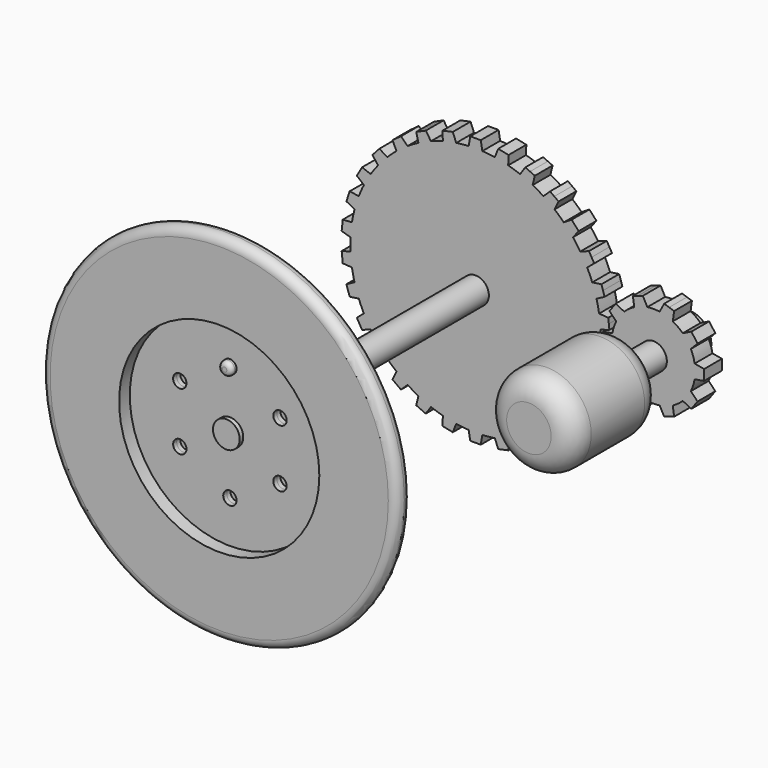
from build123d import *

# Parameters (mm, degrees)
F0_R      = 3
F1_DEPTH  = 80
F0_R_2    = 5
F2_DEPTH  = 5
F3_DEPTH  = 5
F4_DEPTH  = 25
F6_DEPTH  = 5
F8_DEPTH  = 5
F9_R      = 40
F10_DEPTH = 2
F12_R     = 10
F13_DEPTH = 25
F16_R     = 25
F17_DEPTH = 2
F19_R     = 22.5
F20_DEPTH = 3
F21_R     = 1.5
F22_DEPTH = 2
F23_DEPTH = 3.5
F24_R     = 1
F25_R     = 1.99999
F26_R     = 5


# Not quite as in the source:
# - a fillet or chamfer is up to 0.001 mm smaller than in the source, because OpenCascade refuses the exact size
# - a feature of the source that left no trace in its solid (it failed there, or was rolled back) is left out


with BuildPart() as f1:
    # F0 (on Front) → F1 (new body)
    with BuildSketch(Plane.XZ):
        Circle(F0_R)
    extrude(amount=F1_DEPTH)

    # F5 (on face) → F6 (join)
    with BuildSketch(Plane.XZ.offset(5)):
        with BuildLine():
            ThreePointArc((28.0898484802, -1.4057159597), (28.1162107467, -0.7030776964), (28.125, 0))
            ThreePointArc((28.125, 0), (28.1162107467, 0.7030776964), (28.0898484802, 1.4057159597))
            ThreePointArc((28.0898484802, 1.4057159597), (27.9709283072, 2.9398630294), (27.7682826779, 4.4652101991))
            ThreePointArc((27.7682826779, 4.4652101991), (27.5104012706, 5.8475163042), (27.1837531139, 7.2152055856))
            ThreePointArc((27.1837531139, 7.2152055856), (26.7484645208, 8.6911029668), (26.2331096755, 10.1409852457))
            ThreePointArc((26.2331096755, 10.1409852457), (25.6934659962, 11.4394680865), (25.0895972944, 12.709356105))
            ThreePointArc((25.0895972944, 12.709356105), (24.3569644814, 14.0625), (23.5514238999, 15.3735505752))
            ThreePointArc((23.5514238999, 15.3735505752), (22.7536029668, 16.5314602207), (21.8989056799, 17.6480467764))
            ThreePointArc((21.8989056799, 17.6480467764), (20.9009482166, 18.8192983038), (19.8404278876, 19.934217974))
            ThreePointArc((19.8404278876, 19.934217974), (18.8192983038, 20.9009482166), (17.7511268046, 21.815433119))
            ThreePointArc((17.7511268046, 21.815433119), (16.5314602207, 22.7536029668), (15.2623099717, 23.6236643925))
            ThreePointArc((15.2623099717, 23.6236643925), (14.0625, 24.3569644814), (12.8275385085, 25.0293803521))
            ThreePointArc((12.8275385085, 25.0293803521), (11.4394680865, 25.6934659962), (10.0171558733, 26.280643318))
            ThreePointArc((10.0171558733, 26.280643318), (8.6911029668, 26.7484645208), (7.3433252263, 27.1494235596))
            ThreePointArc((7.3433252263, 27.1494235596), (5.8475163042, 27.5104012706), (4.3342039956, 27.7890320221))
            ThreePointArc((4.3342039956, 27.7890320221), (2.9398630294, 27.9709283072), (1.5381733945, 28.0829066802))
            ThreePointArc((1.5381733945, 28.0829066802), (0, 28.125), (-1.5381733945, 28.0829066802))
            ThreePointArc((-1.5381733945, 28.0829066802), (-2.9398630294, 27.9709283072), (-4.3342039956, 27.7890320221))
            ThreePointArc((-4.3342039956, 27.7890320221), (-5.8475163042, 27.5104012706), (-7.3433252263, 27.1494235596))
            ThreePointArc((-7.3433252263, 27.1494235596), (-8.6911029668, 26.7484645208), (-10.0171558733, 26.280643318))
            ThreePointArc((-10.0171558733, 26.280643318), (-11.4394680865, 25.6934659962), (-12.8275385085, 25.0293803521))
            ThreePointArc((-12.8275385085, 25.0293803521), (-14.0625, 24.3569644814), (-15.2623099717, 23.6236643925))
            ThreePointArc((-15.2623099717, 23.6236643925), (-16.5314602207, 22.7536029668), (-17.7511268046, 21.815433119))
            ThreePointArc((-17.7511268046, 21.815433119), (-18.8192983038, 20.9009482166), (-19.8404278876, 19.934217974))
            ThreePointArc((-19.8404278876, 19.934217974), (-20.9009482166, 18.8192983038), (-21.8989056799, 17.6480467764))
            ThreePointArc((-21.8989056799, 17.6480467764), (-22.7536029668, 16.5314602207), (-23.5514238999, 15.3735505752))
            ThreePointArc((-23.5514238999, 15.3735505752), (-24.3569644814, 14.0625), (-25.0895972944, 12.709356105))
            ThreePointArc((-25.0895972944, 12.709356105), (-25.6934659962, 11.4394680865), (-26.2331096755, 10.1409852457))
            ThreePointArc((-26.2331096755, 10.1409852457), (-26.7484645208, 8.6911029668), (-27.1837531139, 7.2152055856))
            ThreePointArc((-27.1837531139, 7.2152055856), (-27.5104012706, 5.8475163042), (-27.7682826779, 4.4652101991))
            ThreePointArc((-27.7682826779, 4.4652101991), (-27.9709283072, 2.9398630294), (-28.0898484802, 1.4057159597))
            ThreePointArc((-28.0898484802, 1.4057159597), (-28.125, 0), (-28.0898484802, -1.4057159597))
            ThreePointArc((-28.0898484802, -1.4057159597), (-27.9709283072, -2.9398630294), (-27.7682826779, -4.4652101991))
            ThreePointArc((-27.7682826779, -4.4652101991), (-27.5104012706, -5.8475163042), (-27.1837531139, -7.2152055856))
            ThreePointArc((-27.1837531139, -7.2152055856), (-26.7484645208, -8.6911029668), (-26.2331096755, -10.1409852457))
            ThreePointArc((-26.2331096755, -10.1409852457), (-25.6934659962, -11.4394680865), (-25.0895972944, -12.709356105))
            ThreePointArc((-25.0895972944, -12.709356105), (-24.3569644814, -14.0625), (-23.5514238999, -15.3735505752))
            ThreePointArc((-23.5514238999, -15.3735505752), (-22.7536029668, -16.5314602207), (-21.8989056799, -17.6480467764))
            ThreePointArc((-21.8989056799, -17.6480467764), (-20.9009482166, -18.8192983038), (-19.8404278876, -19.934217974))
            ThreePointArc((-19.8404278876, -19.934217974), (-18.8192983038, -20.9009482166), (-17.7511268046, -21.815433119))
            ThreePointArc((-17.7511268046, -21.815433119), (-16.5314602207, -22.7536029668), (-15.2623099717, -23.6236643925))
            ThreePointArc((-15.2623099717, -23.6236643925), (-14.0625, -24.3569644814), (-12.8275385085, -25.0293803521))
            ThreePointArc((-12.8275385085, -25.0293803521), (-11.4394680865, -25.6934659962), (-10.0171558733, -26.280643318))
            ThreePointArc((-10.0171558733, -26.280643318), (-8.6911029668, -26.7484645208), (-7.3433252263, -27.1494235596))
            ThreePointArc((-7.3433252263, -27.1494235596), (-5.8475163042, -27.5104012706), (-4.3342039956, -27.7890320221))
            ThreePointArc((-4.3342039956, -27.7890320221), (-2.9398630294, -27.9709283072), (-1.5381733945, -28.0829066802))
            ThreePointArc((-1.5381733945, -28.0829066802), (0, -28.125), (1.5381733945, -28.0829066802))
            ThreePointArc((1.5381733945, -28.0829066802), (2.9398630294, -27.9709283072), (4.3342039956, -27.7890320221))
            ThreePointArc((4.3342039956, -27.7890320221), (5.8475163042, -27.5104012706), (7.3433252263, -27.1494235596))
            ThreePointArc((7.3433252263, -27.1494235596), (8.6911029668, -26.7484645208), (10.0171558733, -26.280643318))
            ThreePointArc((10.0171558733, -26.280643318), (11.4394680865, -25.6934659962), (12.8275385085, -25.0293803521))
            ThreePointArc((12.8275385085, -25.0293803521), (14.0625, -24.3569644814), (15.2623099717, -23.6236643925))
            ThreePointArc((15.2623099717, -23.6236643925), (16.5314602207, -22.7536029668), (17.7511268046, -21.815433119))
            ThreePointArc((17.7511268046, -21.815433119), (18.8192983038, -20.9009482166), (19.8404278876, -19.934217974))
            ThreePointArc((19.8404278876, -19.934217974), (20.9009482166, -18.8192983038), (21.8989056799, -17.6480467764))
            ThreePointArc((21.8989056799, -17.6480467764), (22.7536029668, -16.5314602207), (23.5514238999, -15.3735505752))
            ThreePointArc((23.5514238999, -15.3735505752), (24.3569644814, -14.0625), (25.0895972944, -12.709356105))
            ThreePointArc((25.0895972944, -12.709356105), (25.6934659962, -11.4394680865), (26.2331096755, -10.1409852457))
            ThreePointArc((26.2331096755, -10.1409852457), (26.7484645208, -8.6911029668), (27.1837531139, -7.2152055856))
            ThreePointArc((27.1837531139, -7.2152055856), (27.5104012706, -5.8475163042), (27.7682826779, -4.4652101991))
            ThreePointArc((27.7682826779, -4.4652101991), (27.9709283072, -2.9398630294), (28.0898484802, -1.4057159597))
        make_face()
        with BuildLine():
            ThreePointArc((27.7682826779, 4.4652101991), (27.9709283072, 2.9398630294), (28.0898484802, 1.4057159597))
            Line((28.0898484802, 1.4057159597), (30.0831167926, 1.9772764508))
            Line((30.0831167926, 1.9772764508), (29.959972098, 3.1489199559))
            Line((29.959972098, 3.1489199559), (29.8368274034, 4.3205634611))
            Line((29.8368274034, 4.3205634611), (27.7682826779, 4.4652101991))
        make_face()
        with BuildLine():
            Line((30.0831167926, -1.9772764508), (28.0898484802, -1.4057159597))
            ThreePointArc((28.0898484802, -1.4057159597), (27.9709283072, -2.9398630294), (27.7682826779, -4.4652101991))
            Line((27.7682826779, -4.4652101991), (29.8368274034, -4.3205634611))
            Line((29.8368274034, -4.3205634611), (29.959972098, -3.1489199559))
            Line((29.959972098, -3.1489199559), (30.0831167926, -1.9772764508))
        make_face()
        with BuildLine():
            ThreePointArc((26.2331096755, 10.1409852457), (26.7484645208, 8.6911029668), (27.1837531139, 7.2152055856))
            Line((27.1837531139, 7.2152055856), (29.0146296232, 8.1886998938))
            Line((29.0146296232, 8.1886998938), (28.6505775534, 9.3091369555))
            Line((28.6505775534, 9.3091369555), (28.2865254836, 10.4295740173))
            Line((28.2865254836, 10.4295740173), (26.2331096755, 10.1409852457))
        make_face()
        with BuildLine():
            Line((29.0146296232, -8.1886998938), (27.1837531139, -7.2152055856))
            ThreePointArc((27.1837531139, -7.2152055856), (26.7484645208, -8.6911029668), (26.2331096755, -10.1409852457))
            Line((26.2331096755, -10.1409852457), (28.2865254836, -10.4295740173))
            Line((28.2865254836, -10.4295740173), (28.6505775534, -9.3091369555))
            Line((28.6505775534, -9.3091369555), (29.0146296232, -8.1886998938))
        make_face()
        with BuildLine():
            ThreePointArc((23.5514238999, 15.3735505752), (24.3569644814, 14.0625), (25.0895972944, 12.709356105))
            Line((25.0895972944, 12.709356105), (26.6780639116, 14.0422378576))
            Line((26.6780639116, 14.0422378576), (26.089015289, 15.0625))
            Line((26.089015289, 15.0625), (25.4999666665, 16.0827621424))
            Line((25.4999666665, 16.0827621424), (23.5514238999, 15.3735505752))
        make_face()
        with BuildLine():
            Line((26.6780639116, -14.0422378576), (25.0895972944, -12.709356105))
            ThreePointArc((25.0895972944, -12.709356105), (24.3569644814, -14.0625), (23.5514238999, -15.3735505752))
            Line((23.5514238999, -15.3735505752), (25.4999666665, -16.0827621424))
            Line((25.4999666665, -16.0827621424), (26.089015289, -15.0625))
            Line((26.089015289, -15.0625), (26.6780639116, -14.0422378576))
        make_face()
        with BuildLine():
            ThreePointArc((19.8404278876, 19.934217974), (20.9009482166, 18.8192983038), (21.8989056799, 17.6480467764))
            Line((21.8989056799, 17.6480467764), (23.1755387915, 19.282062645))
            Line((23.1755387915, 19.282062645), (22.3872378675, 20.1575595166))
            Line((22.3872378675, 20.1575595166), (21.5989369435, 21.0330563882))
            Line((21.5989369435, 21.0330563882), (19.8404278876, 19.934217974))
        make_face()
        with BuildLine():
            Line((23.1755387915, -19.282062645), (21.8989056799, -17.6480467764))
            ThreePointArc((21.8989056799, -17.6480467764), (20.9009482166, -18.8192983038), (19.8404278876, -19.934217974))
            Line((19.8404278876, -19.934217974), (21.5989369435, -21.0330563882))
            Line((21.5989369435, -21.0330563882), (22.3872378675, -20.1575595166))
            Line((22.3872378675, -20.1575595166), (23.1755387915, -19.282062645))
        make_face()
        with BuildLine():
            ThreePointArc((15.2623099717, 23.6236643925), (16.5314602207, 22.7536029668), (17.7511268046, 21.815433119))
            Line((17.7511268046, 21.815433119), (18.6601314176, 23.6791687691))
            Line((18.6601314176, 23.6791687691), (17.7070307253, 24.3716369555))
            Line((17.7070307253, 24.3716369555), (16.753930033, 25.064105142))
            Line((16.753930033, 25.064105142), (15.2623099717, 23.6236643925))
        make_face()
        with BuildLine():
            Line((18.6601314176, -23.6791687691), (17.7511268046, -21.815433119))
            ThreePointArc((17.7511268046, -21.815433119), (16.5314602207, -22.7536029668), (15.2623099717, -23.6236643925))
            Line((15.2623099717, -23.6236643925), (16.753930033, -25.064105142))
            Line((16.753930033, -25.064105142), (17.7070307253, -24.3716369555))
            Line((17.7070307253, -24.3716369555), (18.6601314176, -23.6791687691))
        make_face()
        with BuildLine():
            ThreePointArc((10.0171558733, 26.280643318), (11.4394680865, 25.6934659962), (12.8275385085, 25.0293803521))
            Line((12.8275385085, 25.0293803521), (13.3291867596, 27.0413815928))
            Line((13.3291867596, 27.0413815928), (12.2529413727, 27.5205569115))
            Line((12.2529413727, 27.5205569115), (11.1766959857, 27.9997322302))
            Line((11.1766959857, 27.9997322302), (10.0171558733, 26.280643318))
        make_face()
        with BuildLine():
            Line((13.3291867596, -27.0413815928), (12.8275385085, -25.0293803521))
            ThreePointArc((12.8275385085, -25.0293803521), (11.4394680865, -25.6934659962), (10.0171558733, -26.280643318))
            Line((10.0171558733, -26.280643318), (11.1766959857, -27.9997322302))
            Line((11.1766959857, -27.9997322302), (12.2529413727, -27.5205569115))
            Line((12.2529413727, -27.5205569115), (13.3291867596, -27.0413815928))
        make_face()
        with BuildLine():
            ThreePointArc((4.3342039956, 27.7890320221), (5.8475163042, 27.5104012706), (7.3433252263, 27.1494235596))
            Line((7.3433252263, 27.1494235596), (7.4156926796, 29.2217562819))
            Line((7.4156926796, 29.2217562819), (6.2633396859, 29.4666964721))
            Line((6.2633396859, 29.4666964721), (5.1109866922, 29.7116366623))
            Line((5.1109866922, 29.7116366623), (4.3342039956, 27.7890320221))
        make_face()
        with BuildLine():
            Line((7.4156926796, -29.2217562819), (7.3433252263, -27.1494235596))
            ThreePointArc((7.3433252263, -27.1494235596), (5.8475163042, -27.5104012706), (4.3342039956, -27.7890320221))
            Line((4.3342039956, -27.7890320221), (5.1109866922, -29.7116366623))
            Line((5.1109866922, -29.7116366623), (6.2633396859, -29.4666964721))
            Line((6.2633396859, -29.4666964721), (7.4156926796, -29.2217562819))
        make_face()
        with BuildLine():
            ThreePointArc((-1.5381733945, 28.0829066802), (0, 28.125), (1.5381733945, 28.0829066802))
            Line((1.5381733945, 28.0829066802), (1.1780972451, 30.125))
            Line((1.1780972451, 30.125), (0, 30.125))
            Line((0, 30.125), (-1.1780972451, 30.125))
            Line((-1.1780972451, 30.125), (-1.5381733945, 28.0829066802))
        make_face()
        with BuildLine():
            Line((1.1780972451, -30.125), (1.5381733945, -28.0829066802))
            ThreePointArc((1.5381733945, -28.0829066802), (0, -28.125), (-1.5381733945, -28.0829066802))
            Line((-1.5381733945, -28.0829066802), (-1.1780972451, -30.125))
            Line((-1.1780972451, -30.125), (0, -30.125))
            Line((0, -30.125), (1.1780972451, -30.125))
        make_face()
        with BuildLine():
            ThreePointArc((-7.3433252263, 27.1494235596), (-5.8475163042, 27.5104012706), (-4.3342039956, 27.7890320221))
            Line((-4.3342039956, 27.7890320221), (-5.1109866922, 29.7116366623))
            Line((-5.1109866922, 29.7116366623), (-6.2633396859, 29.4666964721))
            Line((-6.2633396859, 29.4666964721), (-7.4156926796, 29.2217562819))
            Line((-7.4156926796, 29.2217562819), (-7.3433252263, 27.1494235596))
        make_face()
        with BuildLine():
            Line((-5.1109866922, -29.7116366623), (-4.3342039956, -27.7890320221))
            ThreePointArc((-4.3342039956, -27.7890320221), (-5.8475163042, -27.5104012706), (-7.3433252263, -27.1494235596))
            Line((-7.3433252263, -27.1494235596), (-7.4156926796, -29.2217562819))
            Line((-7.4156926796, -29.2217562819), (-6.2633396859, -29.4666964721))
            Line((-6.2633396859, -29.4666964721), (-5.1109866922, -29.7116366623))
        make_face()
        with BuildLine():
            ThreePointArc((-12.8275385085, 25.0293803521), (-11.4394680865, 25.6934659962), (-10.0171558733, 26.280643318))
            Line((-10.0171558733, 26.280643318), (-11.1766959857, 27.9997322302))
            Line((-11.1766959857, 27.9997322302), (-12.2529413727, 27.5205569115))
            Line((-12.2529413727, 27.5205569115), (-13.3291867596, 27.0413815928))
            Line((-13.3291867596, 27.0413815928), (-12.8275385085, 25.0293803521))
        make_face()
        with BuildLine():
            Line((-11.1766959857, -27.9997322302), (-10.0171558733, -26.280643318))
            ThreePointArc((-10.0171558733, -26.280643318), (-11.4394680865, -25.6934659962), (-12.8275385085, -25.0293803521))
            Line((-12.8275385085, -25.0293803521), (-13.3291867596, -27.0413815928))
            Line((-13.3291867596, -27.0413815928), (-12.2529413727, -27.5205569115))
            Line((-12.2529413727, -27.5205569115), (-11.1766959857, -27.9997322302))
        make_face()
        with BuildLine():
            ThreePointArc((-17.7511268046, 21.815433119), (-16.5314602207, 22.7536029668), (-15.2623099717, 23.6236643925))
            Line((-15.2623099717, 23.6236643925), (-16.753930033, 25.064105142))
            Line((-16.753930033, 25.064105142), (-17.7070307253, 24.3716369555))
            Line((-17.7070307253, 24.3716369555), (-18.6601314176, 23.6791687691))
            Line((-18.6601314176, 23.6791687691), (-17.7511268046, 21.815433119))
        make_face()
        with BuildLine():
            Line((-16.753930033, -25.064105142), (-15.2623099717, -23.6236643925))
            ThreePointArc((-15.2623099717, -23.6236643925), (-16.5314602207, -22.7536029668), (-17.7511268046, -21.815433119))
            Line((-17.7511268046, -21.815433119), (-18.6601314176, -23.6791687691))
            Line((-18.6601314176, -23.6791687691), (-17.7070307253, -24.3716369555))
            Line((-17.7070307253, -24.3716369555), (-16.753930033, -25.064105142))
        make_face()
        with BuildLine():
            ThreePointArc((-21.8989056799, 17.6480467764), (-20.9009482166, 18.8192983038), (-19.8404278876, 19.934217974))
            Line((-19.8404278876, 19.934217974), (-21.5989369435, 21.0330563882))
            Line((-21.5989369435, 21.0330563882), (-22.3872378675, 20.1575595166))
            Line((-22.3872378675, 20.1575595166), (-23.1755387915, 19.282062645))
            Line((-23.1755387915, 19.282062645), (-21.8989056799, 17.6480467764))
        make_face()
        with BuildLine():
            Line((-21.5989369435, -21.0330563882), (-19.8404278876, -19.934217974))
            ThreePointArc((-19.8404278876, -19.934217974), (-20.9009482166, -18.8192983038), (-21.8989056799, -17.6480467764))
            Line((-21.8989056799, -17.6480467764), (-23.1755387915, -19.282062645))
            Line((-23.1755387915, -19.282062645), (-22.3872378675, -20.1575595166))
            Line((-22.3872378675, -20.1575595166), (-21.5989369435, -21.0330563882))
        make_face()
        with BuildLine():
            ThreePointArc((-25.0895972944, 12.709356105), (-24.3569644814, 14.0625), (-23.5514238999, 15.3735505752))
            Line((-23.5514238999, 15.3735505752), (-25.4999666665, 16.0827621424))
            Line((-25.4999666665, 16.0827621424), (-26.089015289, 15.0625))
            Line((-26.089015289, 15.0625), (-26.6780639116, 14.0422378576))
            Line((-26.6780639116, 14.0422378576), (-25.0895972944, 12.709356105))
        make_face()
        with BuildLine():
            Line((-25.4999666665, -16.0827621424), (-23.5514238999, -15.3735505752))
            ThreePointArc((-23.5514238999, -15.3735505752), (-24.3569644814, -14.0625), (-25.0895972944, -12.709356105))
            Line((-25.0895972944, -12.709356105), (-26.6780639116, -14.0422378576))
            Line((-26.6780639116, -14.0422378576), (-26.089015289, -15.0625))
            Line((-26.089015289, -15.0625), (-25.4999666665, -16.0827621424))
        make_face()
        with BuildLine():
            ThreePointArc((-27.1837531139, 7.2152055856), (-26.7484645208, 8.6911029668), (-26.2331096755, 10.1409852457))
            Line((-26.2331096755, 10.1409852457), (-28.2865254836, 10.4295740173))
            Line((-28.2865254836, 10.4295740173), (-28.6505775534, 9.3091369555))
            Line((-28.6505775534, 9.3091369555), (-29.0146296232, 8.1886998938))
            Line((-29.0146296232, 8.1886998938), (-27.1837531139, 7.2152055856))
        make_face()
        with BuildLine():
            Line((-28.2865254836, -10.4295740173), (-26.2331096755, -10.1409852457))
            ThreePointArc((-26.2331096755, -10.1409852457), (-26.7484645208, -8.6911029668), (-27.1837531139, -7.2152055856))
            Line((-27.1837531139, -7.2152055856), (-29.0146296232, -8.1886998938))
            Line((-29.0146296232, -8.1886998938), (-28.6505775534, -9.3091369555))
            Line((-28.6505775534, -9.3091369555), (-28.2865254836, -10.4295740173))
        make_face()
        with BuildLine():
            ThreePointArc((-28.0898484802, 1.4057159597), (-27.9709283072, 2.9398630294), (-27.7682826779, 4.4652101991))
            Line((-27.7682826779, 4.4652101991), (-29.8368274034, 4.3205634611))
            Line((-29.8368274034, 4.3205634611), (-29.959972098, 3.1489199559))
            Line((-29.959972098, 3.1489199559), (-30.0831167926, 1.9772764508))
            Line((-30.0831167926, 1.9772764508), (-28.0898484802, 1.4057159597))
        make_face()
        with BuildLine():
            Line((-29.8368274034, -4.3205634611), (-27.7682826779, -4.4652101991))
            ThreePointArc((-27.7682826779, -4.4652101991), (-27.9709283072, -2.9398630294), (-28.0898484802, -1.4057159597))
            Line((-28.0898484802, -1.4057159597), (-30.0831167926, -1.9772764508))
            Line((-30.0831167926, -1.9772764508), (-29.959972098, -3.1489199559))
            Line((-29.959972098, -3.1489199559), (-29.8368274034, -4.3205634611))
        make_face()
    extrude(amount=F6_DEPTH)


with BuildPart() as f2:
    # F0 (on Front) → F2 (new body)
    with BuildSketch(Plane.XZ):
        Circle(F0_R_2)
        Circle(F0_R, mode=Mode.SUBTRACT)
    extrude(amount=F2_DEPTH)


with BuildPart() as f3:
    # F0 (on Front) → F3 (new body)
    with BuildSketch(Plane.XZ):
        with Locations((40, 0)):
            Circle(F0_R_2)
        with Locations((40, 0)):
            Circle(F0_R, mode=Mode.SUBTRACT)
    extrude(amount=F3_DEPTH)


with BuildPart() as f4:
    # F0 (on Front) → F4 (new body)
    with BuildSketch(Plane.XZ):
        with Locations((40, 0)):
            Circle(F0_R)
    extrude(amount=F4_DEPTH)

    # F7 (on face) → F8 (join)
    with BuildSketch(Plane.XZ.offset(5)):
        with BuildLine():
            ThreePointArc((49.2453733036, -1.5536078905), (49.3425371212, -0.7795031363), (49.375, 0))
            ThreePointArc((49.375, 0), (49.3425371212, 0.7795031363), (49.2453733036, 1.5536078905))
            ThreePointArc((49.2453733036, 1.5536078905), (48.9161548403, 2.8970343223), (48.3928519278, 4.1773988938))
            ThreePointArc((48.3928519278, 4.1773988938), (47.5845343223, 5.5104867402), (46.566476316, 6.6911892658))
            ThreePointArc((46.566476316, 6.6911892658), (45.5104867402, 7.5845343223), (44.3345463782, 8.3127812852))
            ThreePointArc((44.3345463782, 8.3127812852), (42.8970343223, 8.9161548403), (41.3794085621, 9.2729637667))
            ThreePointArc((41.3794085621, 9.2729637667), (40, 9.375), (38.6205914379, 9.2729637667))
            ThreePointArc((38.6205914379, 9.2729637667), (37.1029656777, 8.9161548403), (35.6654536218, 8.3127812852))
            ThreePointArc((35.6654536218, 8.3127812852), (34.4895132598, 7.5845343223), (33.433523684, 6.6911892658))
            ThreePointArc((33.433523684, 6.6911892658), (32.4154656777, 5.5104867402), (31.6071480722, 4.1773988938))
            ThreePointArc((31.6071480722, 4.1773988938), (31.0838451597, 2.8970343223), (30.7546266964, 1.5536078905))
            ThreePointArc((30.7546266964, 1.5536078905), (30.625, 0), (30.7546266964, -1.5536078905))
            ThreePointArc((30.7546266964, -1.5536078905), (31.0838451597, -2.8970343223), (31.6071480722, -4.1773988938))
            ThreePointArc((31.6071480722, -4.1773988938), (32.4154656777, -5.5104867402), (33.433523684, -6.6911892658))
            ThreePointArc((33.433523684, -6.6911892658), (34.4895132598, -7.5845343223), (35.6654536218, -8.3127812852))
            ThreePointArc((35.6654536218, -8.3127812852), (37.1029656777, -8.9161548403), (38.6205914379, -9.2729637667))
            ThreePointArc((38.6205914379, -9.2729637667), (40, -9.375), (41.3794085621, -9.2729637667))
            ThreePointArc((41.3794085621, -9.2729637667), (42.8970343223, -8.9161548403), (44.3345463782, -8.3127812852))
            ThreePointArc((44.3345463782, -8.3127812852), (45.5104867402, -7.5845343223), (46.566476316, -6.6911892658))
            ThreePointArc((46.566476316, -6.6911892658), (47.5845343223, -5.5104867402), (48.3928519278, -4.1773988938))
            ThreePointArc((48.3928519278, -4.1773988938), (48.9161548403, -2.8970343223), (49.2453733036, -1.5536078905))
        make_face()
        with BuildLine():
            ThreePointArc((49.2453733036, 1.5536078905), (49.3425371212, 0.7795031363), (49.375, 0))
            ThreePointArc((49.375, 0), (49.3425371212, -0.7795031363), (49.2453733036, -1.5536078905))
            Line((49.2453733036, -1.5536078905), (51.375, -1.1780972451))
            Line((51.375, -1.1780972451), (51.375, 0))
            Line((51.375, 0), (51.375, 1.1780972451))
            Line((51.375, 1.1780972451), (49.2453733036, 1.5536078905))
        make_face()
        with BuildLine():
            ThreePointArc((46.566476316, 6.6911892658), (47.5845343223, 5.5104867402), (48.3928519278, 4.1773988938))
            Line((48.3928519278, 4.1773988938), (49.8950364974, 5.7329565525))
            Line((49.8950364974, 5.7329565525), (49.202568311, 6.6860572448))
            Line((49.202568311, 6.6860572448), (48.5101001246, 7.6391579371))
            Line((48.5101001246, 7.6391579371), (46.566476316, 6.6911892658))
        make_face()
        with BuildLine():
            Line((49.8950364974, -5.7329565525), (48.3928519278, -4.1773988938))
            ThreePointArc((48.3928519278, -4.1773988938), (47.5845343223, -5.5104867402), (46.566476316, -6.6911892658))
            Line((46.566476316, -6.6911892658), (48.5101001246, -7.6391579371))
            Line((48.5101001246, -7.6391579371), (49.202568311, -6.6860572448))
            Line((49.202568311, -6.6860572448), (49.8950364974, -5.7329565525))
        make_face()
        with BuildLine():
            ThreePointArc((41.3794085621, 9.2729637667), (42.8970343223, 8.9161548403), (44.3345463782, 8.3127812852))
            Line((44.3345463782, 8.3127812852), (44.6355053728, 10.4542158031))
            Line((44.6355053728, 10.4542158031), (43.515068311, 10.8182678729))
            Line((43.515068311, 10.8182678729), (42.3946312492, 11.1823199426))
            Line((42.3946312492, 11.1823199426), (41.3794085621, 9.2729637667))
        make_face()
        with BuildLine():
            Line((44.6355053728, -10.4542158031), (44.3345463782, -8.3127812852))
            ThreePointArc((44.3345463782, -8.3127812852), (42.8970343223, -8.9161548403), (41.3794085621, -9.2729637667))
            Line((41.3794085621, -9.2729637667), (42.3946312492, -11.1823199426))
            Line((42.3946312492, -11.1823199426), (43.515068311, -10.8182678729))
            Line((43.515068311, -10.8182678729), (44.6355053728, -10.4542158031))
        make_face()
        with BuildLine():
            ThreePointArc((35.6654536218, 8.3127812852), (37.1029656777, 8.9161548403), (38.6205914379, 9.2729637667))
            Line((38.6205914379, 9.2729637667), (37.6053687508, 11.1823199426))
            Line((37.6053687508, 11.1823199426), (36.484931689, 10.8182678729))
            Line((36.484931689, 10.8182678729), (35.3644946272, 10.4542158031))
            Line((35.3644946272, 10.4542158031), (35.6654536218, 8.3127812852))
        make_face()
        with BuildLine():
            Line((37.6053687508, -11.1823199426), (38.6205914379, -9.2729637667))
            ThreePointArc((38.6205914379, -9.2729637667), (37.1029656777, -8.9161548403), (35.6654536218, -8.3127812852))
            Line((35.6654536218, -8.3127812852), (35.3644946272, -10.4542158031))
            Line((35.3644946272, -10.4542158031), (36.484931689, -10.8182678729))
            Line((36.484931689, -10.8182678729), (37.6053687508, -11.1823199426))
        make_face()
        with BuildLine():
            ThreePointArc((31.6071480722, 4.1773988938), (32.4154656777, 5.5104867402), (33.433523684, 6.6911892658))
            Line((33.433523684, 6.6911892658), (31.4898998754, 7.6391579371))
            Line((31.4898998754, 7.6391579371), (30.797431689, 6.6860572448))
            Line((30.797431689, 6.6860572448), (30.1049635026, 5.7329565525))
            Line((30.1049635026, 5.7329565525), (31.6071480722, 4.1773988938))
        make_face()
        with BuildLine():
            Line((31.4898998754, -7.6391579371), (33.433523684, -6.6911892658))
            ThreePointArc((33.433523684, -6.6911892658), (32.4154656777, -5.5104867402), (31.6071480722, -4.1773988938))
            Line((31.6071480722, -4.1773988938), (30.1049635026, -5.7329565525))
            Line((30.1049635026, -5.7329565525), (30.797431689, -6.6860572448))
            Line((30.797431689, -6.6860572448), (31.4898998754, -7.6391579371))
        make_face()
        with BuildLine():
            ThreePointArc((30.7546266964, -1.5536078905), (30.625, 0), (30.7546266964, 1.5536078905))
            Line((30.7546266964, 1.5536078905), (28.625, 1.1780972451))
            Line((28.625, 1.1780972451), (28.625, 0))
            Line((28.625, 0), (28.625, -1.1780972451))
            Line((28.625, -1.1780972451), (30.7546266964, -1.5536078905))
        make_face()
    extrude(amount=F8_DEPTH)


with BuildPart() as f10:
    # F9 (on face) → F10 (new body, symmetric)
    with BuildSketch(Plane.XZ.offset(80)):
        Circle(F9_R)
    extrude(amount=F10_DEPTH, both=True)

    # F11: cut F1
    add(f1.part, mode=Mode.SUBTRACT)

    # F19 (on face) → F20 (cut)
    with BuildSketch(Plane.XZ.offset(82)):
        Circle(F19_R)
    extrude(amount=-F20_DEPTH, mode=Mode.SUBTRACT)


with BuildPart() as f13:
    # F12 (on face) → F13 (new body)
    with BuildSketch(Plane.XZ.offset(25)):
        with Locations((40, 0)):
            Circle(F12_R)
    extrude(amount=F13_DEPTH)


with BuildPart() as f13_1:
    # F14: moved
    add(f13.part.moved(Location((0, 5, 0))))

    # F15: cut F4
    add(f4.part, mode=Mode.SUBTRACT)

    # F26
    f26_edges = [f13_1.edges().sort_by_distance(p)[0] for p in [
        (30, -45, 0),
        (30, -20, 0),
    ]]
    fillet(f26_edges, radius=F26_R)


with BuildPart() as f17:
    # F16 (on face) → F17 (new body)
    with BuildSketch(Plane(origin=(0, -78, 0), x_dir=(-1, 0, 0), z_dir=(0, 1, 0))):
        Circle(F16_R)
    extrude(amount=F17_DEPTH)

    # F18: cut F1
    add(f1.part, mode=Mode.SUBTRACT)


with BuildPart() as f22_tool:
    # F21 (on face) → F22 (new body)
    with BuildSketch(Plane.XZ.offset(79)):
        with Locations((0, 13)):
            Circle(F21_R)
        with Locations((-11.2583302492, 6.5)):
            Circle(F21_R)
        with Locations((-11.2583302492, -6.5)):
            Circle(F21_R)
        with Locations((0, -13)):
            Circle(F21_R)
        with Locations((11.2583302492, -6.5)):
            Circle(F21_R)
        with Locations((11.2583302492, 6.5)):
            Circle(F21_R)
    extrude(amount=-F22_DEPTH)


with BuildPart() as f10_1:
    add(f10.part)

    # F22: cut by f22_tool
    add(f22_tool.part, mode=Mode.SUBTRACT)

    # F25 (radius 2 in the source; OpenCascade refuses exactly that, so slightly less here)
    f25_edges = [f10_1.edges().sort_by_distance(p)[0] for p in [
        (-40, -82, 0),
        (-40, -78, 0),
    ]]
    fillet(f25_edges, radius=F25_R)


with BuildPart() as f17_1:
    add(f17.part)

    # F22: cut by f22_tool
    add(f22_tool.part, mode=Mode.SUBTRACT)


with BuildPart() as f23:
    # F23 (new): a face of the model
    f23_faces = [f17_1.part.faces().sort_by_distance(p)[0] for p in [
        (0, -77, 13),
    ]]
    extrude(f23_faces, amount=F23_DEPTH)

    # F24
    f24_edges = [f23.edges().sort_by_distance(p)[0] for p in [
        (-1.5, -80.5, 13),
    ]]
    fillet(f24_edges, radius=F24_R)


solid = Compound([f1.part, f2.part, f3.part, f4.part, f13_1.part, f10_1.part, f17_1.part, f23.part])
